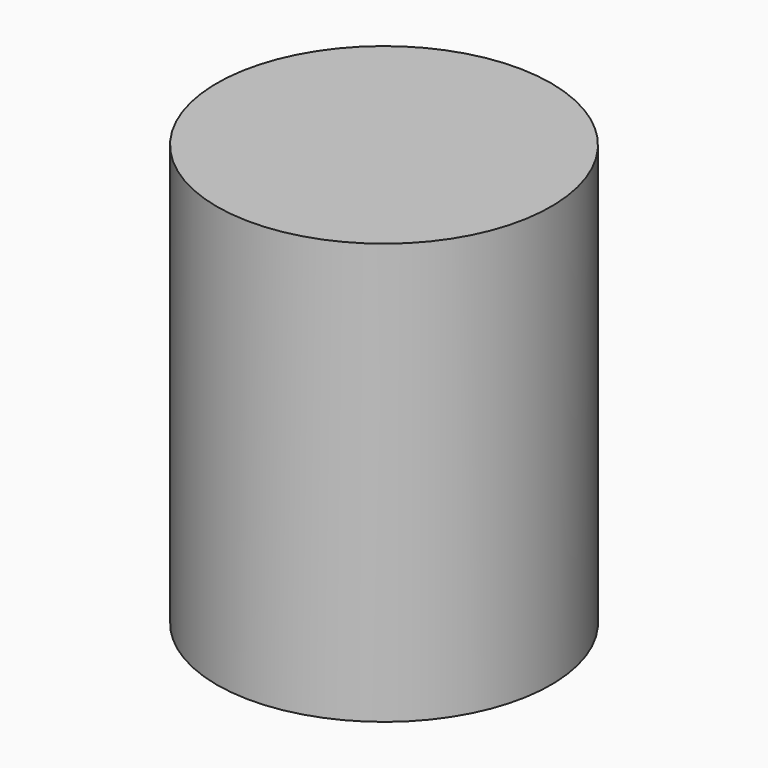
from build123d import *

# Parameters (mm, degrees)
F1_DEPTH = 750


# Not quite as in the source:
# - a feature of the source that left no trace in its solid (it failed there, or was rolled back) is left out


with BuildPart() as f1:
    # F0 (on Top) → F1 (new body)
    with BuildSketch(Plane.XY):
        with BuildLine():
            ThreePointArc((283.1559480312, 92.0029446208), (175, 240.8668360825), (0, 297.7277829232))
            Line((0, 297.7277829232), (283.1559480312, 92.0029446208))
        make_face()
        Polygon((283.1559480312, 92.0029446208), (0, 297.7277829232), (-283.1559480312, 92.0029446208), (-175, -240.8668360825), (175, -240.8668360825), align=None)
        with BuildLine():
            Line((-283.1559480312, 92.0029446208), (0, 297.7277829232))
            ThreePointArc((0, 297.7277829232), (-175, 240.8668360825), (-283.1559480312, 92.0029446208))
        make_face()
        with BuildLine():
            ThreePointArc((297.7277829232, 0), (294.0622598645, 46.5748864492), (283.1559480312, 92.0029446208))
            Line((283.1559480312, 92.0029446208), (175, -240.8668360825))
            ThreePointArc((175, -240.8668360825), (265.2773970167, -135.1655849557), (297.7277829232, 0))
        make_face()
        with BuildLine():
            Line((-175, -240.8668360825), (-283.1559480312, 92.0029446208))
            ThreePointArc((-283.1559480312, 92.0029446208), (-283.1559480312, -92.0029446208), (-175, -240.8668360825))
        make_face()
        with BuildLine():
            ThreePointArc((-175, -240.8668360825), (0, -297.7277829232), (175, -240.8668360825))
            Line((175, -240.8668360825), (-175, -240.8668360825))
        make_face()
    extrude(amount=-F1_DEPTH)


solid = f1.part
